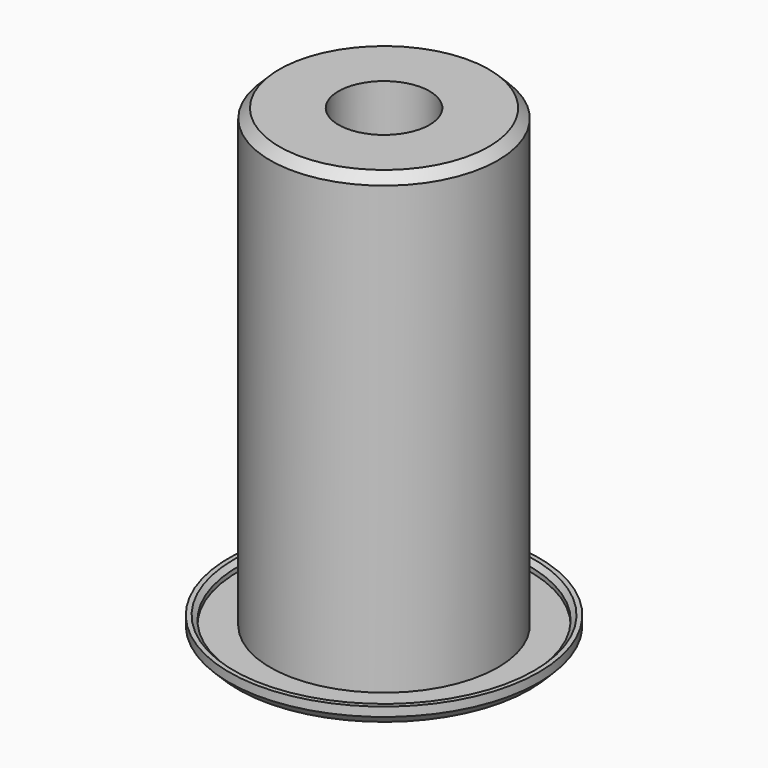
from build123d import *

# Parameters (mm, degrees)
F0_R     = 12.5
F0_R_2   = 6
F0_R_3   = 5
F1_DEPTH = 25
F2_DEPTH = 25
F3_R     = 2
F4_DEPTH = 25
F5_SIZE  = 1
F6_R     = 17
F6_R_2   = 16
F6_R_3   = 12.5
F6_R_4   = 6
F7_DEPTH = 1
F8_DEPTH = 1
F9_SIZE  = 0.5
F10_SIZE = 0.99999


# Not quite as in the source:
# - a fillet or chamfer is up to 0.001 mm smaller than in the source, because OpenCascade refuses the exact size


with BuildPart() as f1:
    # F0 (on Top) → F1 (new body)
    with BuildSketch(Plane.XY):
        Circle(F0_R)
        Circle(F0_R_2, mode=Mode.SUBTRACT)
        Circle(F0_R_2)
        Circle(F0_R_3, mode=Mode.SUBTRACT)
    extrude(amount=F1_DEPTH)

    # F0 (on Top) → F2 (join)
    with BuildSketch(Plane.XY):
        Circle(F0_R)
        Circle(F0_R_2, mode=Mode.SUBTRACT)
    extrude(amount=-F2_DEPTH)

    # F3 (on Right) → F4 (cut)
    with BuildSketch(Plane.YZ):
        with Locations((0, -18)):
            Circle(F3_R)
        with Locations((0, -10)):
            Circle(F3_R)
        with Locations((0, 10)):
            Circle(F3_R)
        with Locations((0, 18)):
            Circle(F3_R)
    extrude(amount=-F4_DEPTH, mode=Mode.SUBTRACT)

    # F5
    f5_edges = [f1.edges().sort_by_distance(p)[0] for p in [
        (-12.5, 0, 25),
    ]]
    chamfer(f5_edges, length=F5_SIZE)

    # F6 (on face) → F7 (join)
    with BuildSketch(Plane(origin=(0, 0, -25), x_dir=(1, 0, 0), z_dir=(0, 0, -1))):
        Circle(F6_R)
        Circle(F6_R_2, mode=Mode.SUBTRACT)
        Circle(F6_R_2)
        Circle(F6_R_3, mode=Mode.SUBTRACT)
        Circle(F6_R_3)
        Circle(F6_R_4, mode=Mode.SUBTRACT)
    extrude(amount=F7_DEPTH)

    # F6 (on face) → F8 (join)
    with BuildSketch(Plane(origin=(0, 0, -25), x_dir=(1, 0, 0), z_dir=(0, 0, -1))):
        Circle(F6_R)
        Circle(F6_R_2, mode=Mode.SUBTRACT)
    extrude(amount=-F8_DEPTH)

    # F9
    f9_edges = [f1.edges().sort_by_distance(p)[0] for p in [
        (-16, 0, -24),
    ]]
    chamfer(f9_edges, length=F9_SIZE)

    # F10 (size 1 in the source; OpenCascade refuses exactly that, so slightly less here)
    f10_edges = [f1.edges().sort_by_distance(p)[0] for p in [
        (-17, 0, -26),
    ]]
    chamfer(f10_edges, length=F10_SIZE)


solid = f1.part
